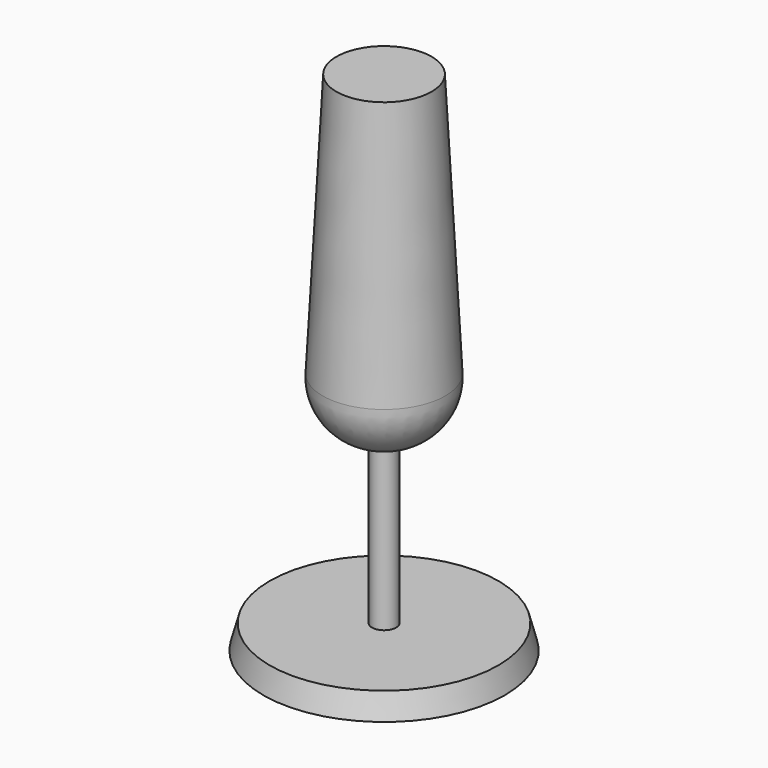
from build123d import *

# Parameters (mm, degrees)
F0_R     = 15
F1_DEPTH = 3
F1_TAPER = 15
F2_R     = 1.5
F3_DEPTH = 20
F4_R     = 8
F5_DEPTH = 40
F5_TAPER = 3


# Not quite as in the source:
# - a fillet or chamfer that OpenCascade refuses, or shapes differently, is made with other operations: its cross-section is extruded or revolved along the edge and cut away or added


with BuildPart() as f1:
    # F0 (on Top) → F1 (new body)
    with BuildSketch(Plane.XY):
        Circle(F0_R)
    extrude(amount=F1_DEPTH, taper=F1_TAPER)

    # F2 (on face) → F3 (join)
    with BuildSketch(Plane.XY.offset(3)):
        Circle(F2_R)
    extrude(amount=F3_DEPTH)

    # F4 (on face) → F5 (join)
    with BuildSketch(Plane.XY.offset(23)):
        Circle(F4_R)
    extrude(amount=F5_DEPTH, taper=F5_TAPER)

    # F6: fillet of radius 7 on 1 edges, made by hand

    # F6_s1 → F6_t2 (revolve, cut)
    with BuildSketch(Plane.XZ):
        with BuildLine():
            ThreePointArc((1.5, 23), (5.9953541002, 25.4536811979), (7.6168139169, 30.3116260276))
            Line((7.6168139169, 30.3116260276), (8, 23))
            Line((8, 23), (1.5, 23))
        make_face()
    revolve(axis=Axis((0, 0, 23), (0, 0, -1)), mode=Mode.SUBTRACT)


solid = f1.part
